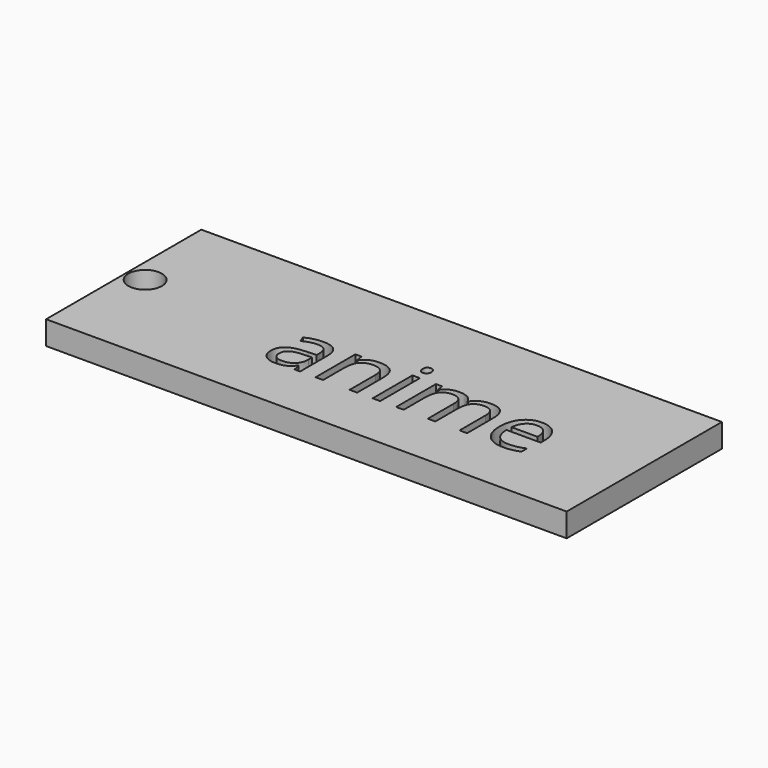
from build123d import *

# Parameters (mm, degrees)
F0_W         = 111.9564399123
F0_H         = 41.7318344116
F1_DEPTH     = 5.08
F2_R         = 3.6061958123
F2_TEXT_SIZE = 19.9865122947
F3_DEPTH     = 25.4


# Not quite as in the source:
# - Text() gives the source's letters only with a copy of the font that has no kerning and outlines rounded to 1/6400 em; it was checked with that copy


with BuildPart() as f1:
    # F0 (on Top) → F1 (new body)
    with BuildSketch(Plane.XY):
        with Locations((7.9146586359, 1.8707364798)):
            Rectangle(F0_W, F0_H)
    extrude(amount=F1_DEPTH)

    # F2 (on face) → F3 (cut)
    with BuildSketch(Plane.XY.offset(5.08)):
        with Locations((-44.0342798829, 2.5902516209)):
            Circle(F2_R)
        with Locations((-12.3756472021, -7.1951444261)):
            Text('anime', F2_TEXT_SIZE, font='Open Sans', text_align=(TextAlign.LEFT, TextAlign.BOTTOM))
    extrude(amount=-F3_DEPTH, mode=Mode.SUBTRACT)


solid = f1.part
